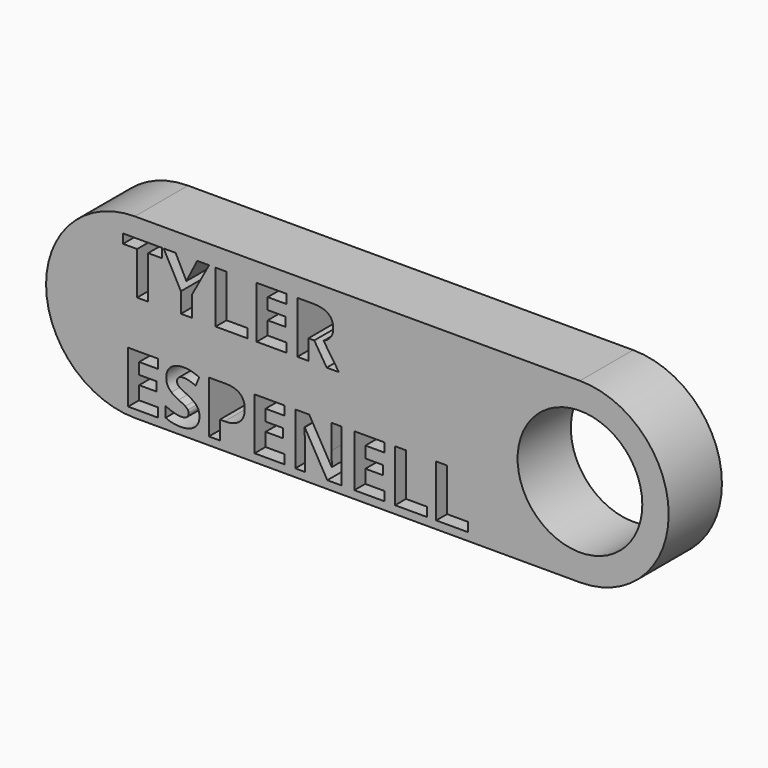
from build123d import *

# Parameters (mm, degrees)
F0_R     = 14.055422355
F1_DEPTH = 15


with BuildPart() as f1:
    # F0 (on Front) → F1 (new body)
    with BuildSketch(Plane.XZ):
        with BuildLine():
            Line((40.1303427248, 20), (-60.1955140871, 20))
            ThreePointArc((-60.1955140871, 20), (-80.1955140871, 0), (-60.1955140871, -20))
            Line((-60.1955140871, -20), (40.1303427248, -20))
            ThreePointArc((40.1303427248, -20), (60.1303427248, 0), (40.1303427248, 20))
        make_face()
        Polygon((-54.9684894893, -16.192931808), (-54.9684894893, -18.2415492212), (-61.705880007, -18.2415492212), (-61.705880007, -6.5413830201), (-54.9684894893, -6.5413830201), (-54.9684894893, -8.5746358027), (-59.2244921653, -8.5746358027), (-59.2244921653, -11.1430898845), (-55.2629782425, -11.1430898845), (-55.2629782425, -13.1763426671), (-59.2244921653, -13.1763426671), (-59.2244921653, -16.192931808), align=None, mode=Mode.SUBTRACT)
        with BuildLine():
            add(Edge.make_bspline(
                [(-46.2298558362, -13.0598275517), (-45.6216725417, -13.8472648699), (-45.6216725417, -14.9919298495)],
                knots=[0, 0, 0, 1, 1, 1], degree=2))
            add(Edge.make_bspline(
                [(-45.6216725417, -14.9919298495), (-45.6216725417, -16.577047573), (-46.7624963636, -17.4899627077)],
                knots=[0, 0, 0, 1, 1, 1], degree=2))
            add(Edge.make_bspline(
                [(-46.7624963636, -17.4899627077), (-47.9033201856, -18.4028778425), (-49.9340121964, -18.4028778425)],
                knots=[0, 0, 0, 1, 1, 1], degree=2))
            add(Edge.make_bspline(
                [(-49.9340121964, -18.4028778425), (-51.8084971295, -18.4028778425), (-53.2476508623, -17.6961048349)],
                knots=[0, 0, 0, 1, 1, 1], degree=2))
            Line((-53.2476508623, -17.6961048349), (-53.2476508623, -15.3914102451))
            add(Edge.make_bspline(
                [(-53.2476508623, -15.3914102451), (-52.0645743062, -15.9214900007), (-51.243846955, -16.1365948291)],
                knots=[0, 0, 0, 1, 1, 1], degree=2))
            add(Edge.make_bspline(
                [(-51.243846955, -16.1365948291), (-50.4231196038, -16.3516996575), (-49.7419543139, -16.3516996575)],
                knots=[0, 0, 0, 1, 1, 1], degree=2))
            add(Edge.make_bspline(
                [(-49.7419543139, -16.3516996575), (-48.9276288922, -16.3516996575), (-48.491017306, -16.0405658879)],
                knots=[0, 0, 0, 1, 1, 1], degree=2))
            add(Edge.make_bspline(
                [(-48.491017306, -16.0405658879), (-48.0544057198, -15.7294321183), (-48.0544057198, -15.1122861225)],
                knots=[0, 0, 0, 1, 1, 1], degree=2))
            add(Edge.make_bspline(
                [(-48.0544057198, -15.1122861225), (-48.0544057198, -14.7691427058), (-48.2464636023, -14.5002616703)],
                knots=[0, 0, 0, 1, 1, 1], degree=2))
            add(Edge.make_bspline(
                [(-48.2464636023, -14.5002616703), (-48.4385214848, -14.2313806349), (-48.8111137768, -13.9842661594)],
                knots=[0, 0, 0, 1, 1, 1], degree=2))
            add(Edge.make_bspline(
                [(-48.8111137768, -13.9842661594), (-49.1837060689, -13.7371516839), (-50.3283710485, -13.1917072977)],
                knots=[0, 0, 0, 1, 1, 1], degree=2))
            add(Edge.make_bspline(
                [(-50.3283710485, -13.1917072977), (-51.3987736469, -12.6872352597), (-51.9352553319, -12.2237355699)],
                knots=[0, 0, 0, 1, 1, 1], degree=2))
            add(Edge.make_bspline(
                [(-51.9352553319, -12.2237355699), (-52.471737017, -11.7602358802), (-52.7918334878, -11.1430898845)],
                knots=[0, 0, 0, 1, 1, 1], degree=2))
            add(Edge.make_bspline(
                [(-52.7918334878, -11.1430898845), (-53.1119299586, -10.5259438888), (-53.1119299586, -9.7039361517)],
                knots=[0, 0, 0, 1, 1, 1], degree=2))
            add(Edge.make_bspline(
                [(-53.1119299586, -9.7039361517), (-53.1119299586, -8.1495476895), (-52.0594527626, -7.2622402724)],
                knots=[0, 0, 0, 1, 1, 1], degree=2))
            add(Edge.make_bspline(
                [(-52.0594527626, -7.2622402724), (-51.0069755666, -6.3749328553), (-49.1504160359, -6.3749328553)],
                knots=[0, 0, 0, 1, 1, 1], degree=2))
            add(Edge.make_bspline(
                [(-49.1504160359, -6.3749328553), (-48.238781287, -6.3749328553), (-47.4103716206, -6.5900376837)],
                knots=[0, 0, 0, 1, 1, 1], degree=2))
            add(Edge.make_bspline(
                [(-47.4103716206, -6.5900376837), (-46.5819619541, -6.805142512), (-45.6780095205, -7.1969405923)],
                knots=[0, 0, 0, 1, 1, 1], degree=2))
            Line((-45.6780095205, -7.1969405923), (-46.4769703117, -9.1277625042))
            add(Edge.make_bspline(
                [(-46.4769703117, -9.1277625042), (-47.4142127782, -8.7436467393), (-48.0262372304, -8.5912808192)],
                knots=[0, 0, 0, 1, 1, 1], degree=2))
            add(Edge.make_bspline(
                [(-48.0262372304, -8.5912808192), (-48.6382616826, -8.4389148991), (-49.2297999607, -8.4389148991)],
                knots=[0, 0, 0, 1, 1, 1], degree=2))
            add(Edge.make_bspline(
                [(-49.2297999607, -8.4389148991), (-49.9340121964, -8.4389148991), (-50.3104456461, -8.7666936852)],
                knots=[0, 0, 0, 1, 1, 1], degree=2))
            add(Edge.make_bspline(
                [(-50.3104456461, -8.7666936852), (-50.6868790958, -9.0944724713), (-50.6868790958, -9.6219914552)],
                knots=[0, 0, 0, 1, 1, 1], degree=2))
            add(Edge.make_bspline(
                [(-50.6868790958, -9.6219914552), (-50.6868790958, -9.9497702413), (-50.5345131757, -10.194323945)],
                knots=[0, 0, 0, 1, 1, 1], degree=2))
            add(Edge.make_bspline(
                [(-50.5345131757, -10.194323945), (-50.3821472556, -10.4388776487), (-50.0505273118, -10.6667863359)],
                knots=[0, 0, 0, 1, 1, 1], degree=2))
            add(Edge.make_bspline(
                [(-50.0505273118, -10.6667863359), (-49.7189073681, -10.8946950231), (-48.4794938331, -11.4862333012)],
                knots=[0, 0, 0, 1, 1, 1], degree=2))
            add(Edge.make_bspline(
                [(-48.4794938331, -11.4862333012), (-46.8380391308, -12.2723902335), (-46.2298558362, -13.0598275517)],
                knots=[0, 0, 0, 1, 1, 1], degree=2))
        make_face(mode=Mode.SUBTRACT)
        with BuildLine():
            add(Edge.make_bspline(
                [(-36.527091613, -7.4581393125), (-35.419557824, -8.3748956049), (-35.419557824, -10.1904827873)],
                knots=[0, 0, 0, 1, 1, 1], degree=2))
            add(Edge.make_bspline(
                [(-35.419557824, -10.1904827873), (-35.419557824, -12.080332351), (-36.6000736083, -13.0803137258)],
                knots=[0, 0, 0, 1, 1, 1], degree=2))
            add(Edge.make_bspline(
                [(-36.6000736083, -13.0803137258), (-37.7805893927, -14.0802951006), (-39.9572453942, -14.0802951006)],
                knots=[0, 0, 0, 1, 1, 1], degree=2))
            Line((-39.9572453942, -14.0802951006), (-41.0199656773, -14.0802951006))
            Line((-41.0199656773, -14.0802951006), (-41.0199656773, -18.2415492212))
            Line((-41.0199656773, -18.2415492212), (-43.501353519, -18.2415492212))
            Line((-43.501353519, -18.2415492212), (-43.501353519, -6.5413830201))
            Line((-43.501353519, -6.5413830201), (-39.7651875117, -6.5413830201))
            add(Edge.make_bspline(
                [(-39.7651875117, -6.5413830201), (-37.634625402, -6.5413830201), (-36.527091613, -7.4581393125)],
                knots=[0, 0, 0, 1, 1, 1], degree=2))
        make_face(mode=Mode.SUBTRACT)
        Polygon((-26.4722212719, -16.192931808), (-26.4722212719, -18.2415492212), (-33.2096117895, -18.2415492212), (-33.2096117895, -6.5413830201), (-26.4722212719, -6.5413830201), (-26.4722212719, -8.5746358027), (-30.7282239478, -8.5746358027), (-30.7282239478, -11.1430898845), (-26.766710025, -11.1430898845), (-26.766710025, -13.1763426671), (-30.7282239478, -13.1763426671), (-30.7282239478, -16.192931808), align=None, mode=Mode.SUBTRACT)
        with BuildLine():
            Line((-13.6529978088, -6.5413830201), (-13.6529978088, -18.2415492212))
            Line((-13.6529978088, -18.2415492212), (-16.8053078534, -18.2415492212))
            Line((-16.8053078534, -18.2415492212), (-21.8961221252, -9.3915219962))
            Line((-21.8961221252, -9.3915219962), (-21.9678237346, -9.3915219962))
            add(Edge.make_bspline(
                [(-21.9678237346, -9.3915219962), (-21.8141774286, -11.7346281625), (-21.8141774286, -12.7358899232)],
                knots=[0, 0, 0, 1, 1, 1], degree=2))
            Line((-21.8141774286, -12.7358899232), (-21.8141774286, -18.2415492212))
            Line((-21.8141774286, -18.2415492212), (-24.0318057784, -18.2415492212))
            Line((-24.0318057784, -18.2415492212), (-24.0318057784, -6.5413830201))
            Line((-24.0318057784, -6.5413830201), (-20.9025426798, -6.5413830201))
            Line((-20.9025426798, -6.5413830201), (-15.8219714951, -15.304344005))
            Line((-15.8219714951, -15.304344005), (-15.7656345162, -15.304344005))
            add(Edge.make_bspline(
                [(-15.7656345162, -15.304344005), (-15.8859907892, -13.0226963611), (-15.8859907892, -12.080332351)],
                knots=[0, 0, 0, 1, 1, 1], degree=2))
            Line((-15.8859907892, -12.080332351), (-15.8859907892, -6.5413830201))
            Line((-15.8859907892, -6.5413830201), (-13.6529978088, -6.5413830201))
        make_face(mode=Mode.SUBTRACT)
        Polygon((-3.9707197598, -16.192931808), (-3.9707197598, -18.2415492212), (-10.7081102774, -18.2415492212), (-10.7081102774, -6.5413830201), (-3.9707197598, -6.5413830201), (-3.9707197598, -8.5746358027), (-8.2267224357, -8.5746358027), (-8.2267224357, -11.1430898845), (-4.2652085129, -11.1430898845), (-4.2652085129, -13.1763426671), (-8.2267224357, -13.1763426671), (-8.2267224357, -16.192931808), align=None, mode=Mode.SUBTRACT)
        Polygon((5.6961936587, -18.2415492212), (-1.5303042663, -18.2415492212), (-1.5303042663, -6.5413830201), (0.9510835754, -6.5413830201), (0.9510835754, -16.192931808), (5.6961936587, -16.192931808), align=None, mode=Mode.SUBTRACT)
        Polygon((14.9559443664, -18.2415492212), (7.7294464413, -18.2415492212), (7.7294464413, -6.5413830201), (10.2108342831, -6.5413830201), (10.2108342831, -16.192931808), (14.9559443664, -16.192931808), align=None, mode=Mode.SUBTRACT)
        Polygon((-57.1912393827, 13.6835923916), (-57.1912393827, 4.0474082343), (-59.6726272244, 4.0474082343), (-59.6726272244, 13.6835923916), (-62.8505449866, 13.6835923916), (-62.8505449866, 15.7475744354), (-54.0158823922, 15.7475744354), (-54.0158823922, 13.6835923916), align=None, mode=Mode.SUBTRACT)
        Polygon((-50.9992932513, 15.7475744354), (-48.5742423884, 10.9307627426), (-46.133826895, 15.7475744354), (-43.4603811708, 15.7475744354), (-47.3425111687, 8.6004604351), (-47.3425111687, 4.0474082343), (-49.8059736081, 4.0474082343), (-49.8059736081, 8.5210765104), (-53.6881036061, 15.7475744354), align=None, mode=Mode.SUBTRACT)
        Polygon((-34.76143948, 4.0474082343), (-41.987937405, 4.0474082343), (-41.987937405, 15.7475744354), (-39.5065495633, 15.7475744354), (-39.5065495633, 6.0960256475), (-34.76143948, 6.0960256475), align=None, mode=Mode.SUBTRACT)
        Polygon((-25.9907961798, 6.0960256475), (-25.9907961798, 4.0474082343), (-32.7281866974, 4.0474082343), (-32.7281866974, 15.7475744354), (-25.9907961798, 15.7475744354), (-25.9907961798, 13.7143216528), (-30.2467988557, 13.7143216528), (-30.2467988557, 11.145867571), (-26.2852849329, 11.145867571), (-26.2852849329, 9.1126147884), (-30.2467988557, 9.1126147884), (-30.2467988557, 6.0960256475), align=None, mode=Mode.SUBTRACT)
        with BuildLine():
            Line((-19.7501953848, 8.536441141), (-21.0689928446, 8.536441141))
            Line((-21.0689928446, 8.536441141), (-21.0689928446, 4.0474082343))
            Line((-21.0689928446, 4.0474082343), (-23.5503806863, 4.0474082343))
            Line((-23.5503806863, 4.0474082343), (-23.5503806863, 15.7475744354))
            Line((-23.5503806863, 15.7475744354), (-20.1419934651, 15.7475744354))
            add(Edge.make_bspline(
                [(-20.1419934651, 15.7475744354), (-17.7553541788, 15.7475744354), (-16.611969585, 14.8794728066)],
                knots=[0, 0, 0, 1, 1, 1], degree=2))
            add(Edge.make_bspline(
                [(-16.611969585, 14.8794728066), (-15.4685849913, 14.0113711777), (-15.4685849913, 12.2418778871)],
                knots=[0, 0, 0, 1, 1, 1], degree=2))
            add(Edge.make_bspline(
                [(-15.4685849913, 12.2418778871), (-15.4685849913, 11.2098868652), (-16.0357959376, 10.4058045305)],
                knots=[0, 0, 0, 1, 1, 1], degree=2))
            add(Edge.make_bspline(
                [(-16.0357959376, 10.4058045305), (-16.6030068838, 9.6017221958), (-17.6452409928, 9.1459048214)],
                knots=[0, 0, 0, 1, 1, 1], degree=2))
            add(Edge.make_bspline(
                [(-17.6452409928, 9.1459048214), (-15.0025245298, 5.1997555292), (-14.2035637386, 4.0474082343)],
                knots=[0, 0, 0, 1, 1, 1], degree=2))
            Line((-14.2035637386, 4.0474082343), (-16.9563933876, 4.0474082343))
            Line((-16.9563933876, 4.0474082343), (-19.7501953848, 8.536441141))
        make_face(mode=Mode.SUBTRACT)
        with Locations((40.1303427248, 0)):
            Circle(F0_R, mode=Mode.SUBTRACT)
    extrude(amount=F1_DEPTH)


solid = f1.part
